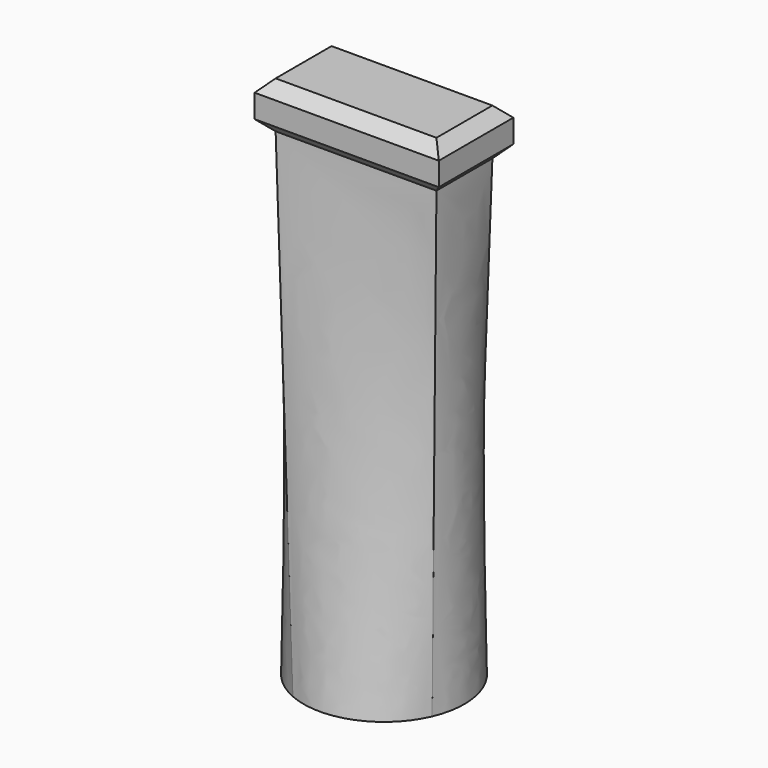
from build123d import *

# Parameters (mm, degrees)
F2_W     = 13.8
F2_H     = 6
F6_W     = 12.6
F6_H     = 4.4
F8_W     = 15.8
F8_H     = 8
F9_DEPTH = 4
F10_SIZE = 0.99999


# Not quite as in the source:
# - a fillet or chamfer is up to 0.001 mm smaller than in the source, because OpenCascade refuses the exact size
# - the arcs of a loft's sections are written as splines that run evenly, so that the points pair up as in the source's solid


with BuildPart() as f3:
    # F0 (on Top) → F3 section 0
    with BuildSketch(Plane.XY):
        with BuildLine():
            add(Edge.make_bspline(
                [(-6.3277833881, 2.7512101688), (-6.6879159571, 1.9229052602), (-6.883211565, 1.0233196176), (-6.914692653, -0.782821821), (-6.7508657466, -1.6886669775), (-6.0887700743, -3.3693713762), (-5.5907618149, -4.143569333), (-4.3358874467, -5.4429646828), (-3.5795150773, -5.9676508192), (-2.7512101688, -6.3277833881)],
                knots=[0, 0, 0, 0, 0.25, 0.25, 0.5, 0.5, 0.75, 0.75, 1, 1, 1, 1], degree=3))
            add(Edge.make_bspline(
                [(-2.7512101688, -6.3277833881), (-1.9229052602, -6.6879159571), (-1.0233196176, -6.883211565), (0.782821821, -6.914692653), (1.6886669775, -6.7508657466), (3.3693713762, -6.0887700743), (4.143569333, -5.5907618149), (5.4429646828, -4.3358874467), (5.9676508192, -3.5795150773), (6.3277833881, -2.7512101688)],
                knots=[0, 0, 0, 0, 0.25, 0.25, 0.5, 0.5, 0.75, 0.75, 1, 1, 1, 1], degree=3))
            add(Edge.make_bspline(
                [(6.3277833881, -2.7512101688), (6.6879159571, -1.9229052602), (6.883211565, -1.0233196176), (6.914692653, 0.782821821), (6.7508657466, 1.6886669775), (6.0887700743, 3.3693713762), (5.5907618149, 4.143569333), (4.3358874467, 5.4429646828), (3.5795150773, 5.9676508192), (2.7512101688, 6.3277833881)],
                knots=[0, 0, 0, 0, 0.25, 0.25, 0.5, 0.5, 0.75, 0.75, 1, 1, 1, 1], degree=3))
            add(Edge.make_bspline(
                [(2.7512101688, 6.3277833881), (1.9229052602, 6.6879159571), (1.0233196176, 6.883211565), (-0.782821821, 6.914692653), (-1.6886669775, 6.7508657466), (-3.3693713762, 6.0887700743), (-4.143569333, 5.5907618149), (-5.4429646828, 4.3358874467), (-5.9676508192, 3.5795150773), (-6.3277833881, 2.7512101688)],
                knots=[0, 0, 0, 0, 0.25, 0.25, 0.5, 0.5, 0.75, 0.75, 1, 1, 1, 1], degree=3))
        make_face()
    # F2 (on offset) → F3 section 1
    with BuildSketch(Plane.XY.offset(40)):
        Rectangle(F2_W, F2_H)
    loft(ruled=True)

    # F5 (on Top) → F7 section 0
    with BuildSketch(Plane.XY):
        with BuildLine():
            add(Edge.make_bspline(
                [(-5.947778016, 2.0770018469), (-6.219656922, 1.2984395252), (-6.3366241137, 0.4661247359), (-6.2431050237, -1.1805579575), (-6.0326555377, -1.9942779624), (-5.3160969794, -3.479826193), (-4.8102698423, -4.151069919), (-3.5797613606, -5.2493224353), (-2.8555641686, -5.6758991101), (-2.0770018469, -5.947778016)],
                knots=[0, 0, 0, 0, 0.25, 0.25, 0.5, 0.5, 0.75, 0.75, 1, 1, 1, 1], degree=3))
            add(Edge.make_bspline(
                [(-2.0770018469, -5.947778016), (-1.2984395252, -6.219656922), (-0.4661247359, -6.3366241137), (1.1805579575, -6.2431050237), (1.9942779624, -6.0326555377), (3.479826193, -5.3160969794), (4.151069919, -4.8102698423), (5.2493224353, -3.5797613606), (5.6758991101, -2.8555641686), (5.947778016, -2.0770018469)],
                knots=[0, 0, 0, 0, 0.25, 0.25, 0.5, 0.5, 0.75, 0.75, 1, 1, 1, 1], degree=3))
            add(Edge.make_bspline(
                [(5.947778016, -2.0770018469), (6.219656922, -1.2984395252), (6.3366241137, -0.4661247359), (6.2431050237, 1.1805579575), (6.0326555377, 1.9942779624), (5.3160969794, 3.479826193), (4.8102698423, 4.151069919), (3.5797613606, 5.2493224353), (2.8555641686, 5.6758991101), (2.0770018469, 5.947778016)],
                knots=[0, 0, 0, 0, 0.25, 0.25, 0.5, 0.5, 0.75, 0.75, 1, 1, 1, 1], degree=3))
            add(Edge.make_bspline(
                [(2.0770018469, 5.947778016), (1.2984395252, 6.219656922), (0.4661247359, 6.3366241137), (-1.1805579575, 6.2431050237), (-1.9942779624, 6.0326555377), (-3.479826193, 5.3160969794), (-4.151069919, 4.8102698423), (-5.2493224353, 3.5797613606), (-5.6758991101, 2.8555641686), (-5.947778016, 2.0770018469)],
                knots=[0, 0, 0, 0, 0.25, 0.25, 0.5, 0.5, 0.75, 0.75, 1, 1, 1, 1], degree=3))
        make_face()
    # F6 (on offset) → F7 section 1
    with BuildSketch(Plane.XY.offset(38)):
        Rectangle(F6_W, F6_H)
    loft(ruled=True, mode=Mode.SUBTRACT)

    # F8 (on offset) → F9 (join)
    with BuildSketch(Plane.XY.offset(40)):
        Rectangle(F8_W, F8_H)
    extrude(amount=F9_DEPTH)

    # F10 (size 1 in the source; OpenCascade refuses exactly that, so slightly less here)
    f10_edges = [f3.edges().sort_by_distance(p)[0] for p in [
        (7.9, 0, 44),
        (0, -4, 44),
        (0, 4, 44),
        (-7.9, 0, 44),
        (0, -4, 40),
        (-7.9, 0, 40),
        (0, 4, 40),
        (7.9, 0, 40),
    ]]
    chamfer(f10_edges, length=F10_SIZE)


solid = f3.part
